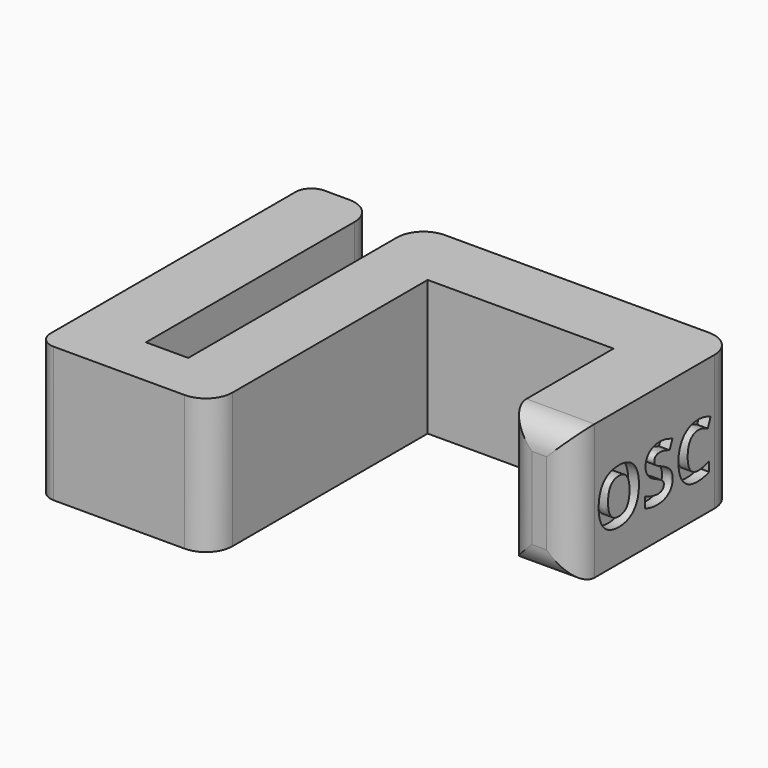
from build123d import *

# Parameters (mm, degrees)
F1_DEPTH     = 25.4
F2_R         = 5
F3_TEXT_SIZE = 20.1439934491
F4_DEPTH     = 2
F5_TEXT_SIZE = 13.9044940261
F6_DEPTH     = 2
F7_R         = 3


# Not quite as in the source:
# - Text() gives the source's letters only with a copy of the font that has no kerning and outlines rounded to 1/6400 em; it was checked with that copy


with BuildPart() as f1:
    # F0 (on Top) → F1 (new body)
    with BuildSketch(Plane.XY):
        Polygon((0, 63.5), (0, 0), (32.5752518936, 0), (32.5752518936, 50.8), (67.4797778515, 50.8), (67.4797778515, 25.3516854542), (80.2734648196, 25.3516854542), (80.2734648196, 63.5), (20.6375, 63.5), (20.6375, 9.52754), (12.7, 9.52754), (12.7, 63.5), align=None)
    extrude(amount=F1_DEPTH)

    # F2
    f2_edges = [f1.edges().sort_by_distance(p)[0] for p in [
        (73.876621, 25.351685, 25.4),
        (73.876621, 25.351685, 0),
        (80.273465, 25.351685, 12.7),
        (67.479778, 25.351685, 12.7),
        (80.273465, 63.5, 12.7),
        (32.575252, 0, 12.7),
        (20.6375, 63.5, 12.7),
        (12.7, 63.5, 12.7),
    ]]
    fillet(f2_edges, radius=F2_R)

    # F3 (on face) → F4 (cut)
    with BuildSketch(Plane(origin=(0, 0, 0), x_dir=(0, -1, 0), z_dir=(-1, 0, 0))):
        with Locations((-52.4805858731, 5.858534711)):
            Text('JEFF', F3_TEXT_SIZE, font='Tinos', text_align=(TextAlign.LEFT, TextAlign.BOTTOM))
    extrude(amount=-F4_DEPTH, mode=Mode.SUBTRACT)

    # F5 (on face) → F6 (cut)
    with BuildSketch(Plane.YZ.offset(80.2734648196)):
        with Locations((30.5019977322, 6.1948261079)):
            Text('OSC', F5_TEXT_SIZE, font='Open Sans', font_style=FontStyle.BOLD, text_align=(TextAlign.LEFT, TextAlign.BOTTOM))
    extrude(amount=-F6_DEPTH, mode=Mode.SUBTRACT)

    # F7
    f7_edges = [f1.edges().sort_by_distance(p)[0] for p in [
        (0, 0, 12.7),
        (0, 63.5, 12.7),
    ]]
    fillet(f7_edges, radius=F7_R)


solid = f1.part
